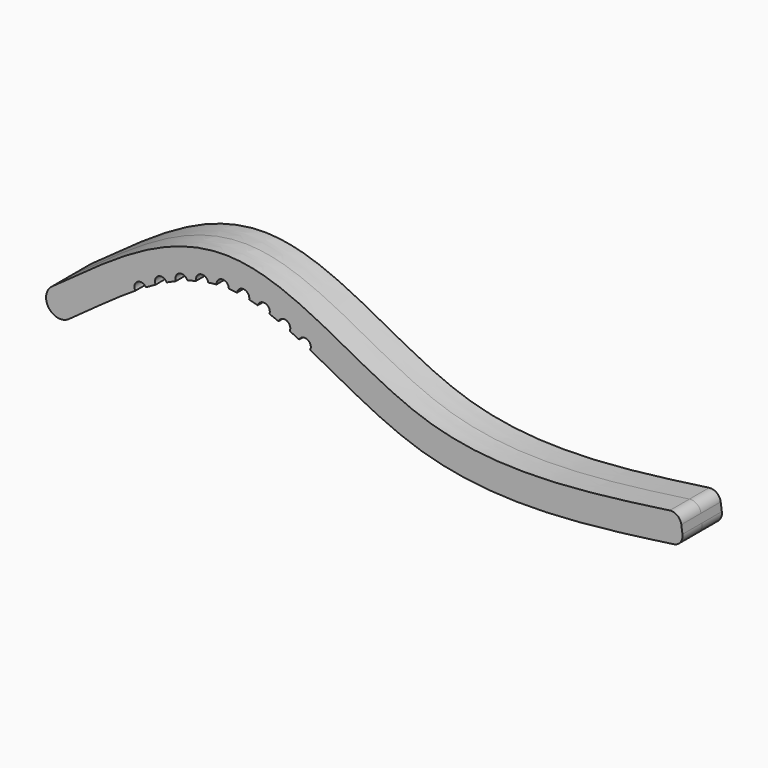
from build123d import *

# Parameters (mm, degrees)
F1_DEPTH = 6
F2_R     = 2.5
F3_R     = 1.5
F4_DEPTH = 12.0010001


# Not quite as in the source:
# - the dataset's text gives a spline's control points without its knots; the knots are read off the source's solid


with BuildPart() as f1:
    # F0 (on Front) → F1 (new body, symmetric)
    with BuildSketch(Plane.XZ):
        with BuildLine():
            ThreePointArc((-4.0449113911, 5.7130282546), (-4.8789698229, 0.8340584318), (0, 0))
            add(Edge.make_bspline(
                [(0, 0), (12.6866183221, 8.9823198273), (39.097046681, 31.0254585121), (84.6231120805, -9.3204370609), (127.451649596, -3.1579744512), (150, 0)],
                knots=[0, 0, 0, 0, 0.3024009423, 0.6287352131, 1, 1, 1, 1], degree=3))
            Line((150, 0), (149.0291016229, 6.9323413319))
            add(Edge.make_bspline(
                [(-4.0449113911, 5.7130282546), (-1.4893265055, 7.522421444), (2.4289578755, 10.3991251109), (7.8311540893, 14.2258677584), (11.985518828, 17.0073967049), (16.2624014486, 19.6143417246), (20.6904437749, 21.9553087459), (25.3048430013, 23.9276125636), (29.3354802395, 25.1619067391), (32.6783528938, 25.828942319), (35.2427144442, 26.1479585874), (37.419626365, 26.2456905562), (39.1857443489, 26.2125714545), (40.9384858731, 26.1049312213), (43.0954900321, 25.8409787708), (46.4720299209, 25.1788075072), (50.5545204313, 23.9683165065), (55.2777949463, 22.0808731164), (59.8806691618, 19.8983979978), (64.4079741748, 17.5399643684), (68.8916038218, 15.1143270568), (73.3515183232, 12.7253635973), (77.7977758185, 10.4736185968), (81.4936492304, 8.7918611912), (84.4432333572, 7.608120023), (86.2840306834, 6.9438576049), (87.7535671011, 6.4632867232), (89.2383433444, 6.0114309597), (91.1197744412, 5.5000916427), (93.4192059549, 4.9686735981), (96.5398637001, 4.3656966777), (100.5419436116, 3.8023805188), (105.4978361754, 3.4066907033), (110.5952082283, 3.2657358671), (117.5618909593, 3.3809979789), (126.5522503494, 4.0218977706), (137.6717582852, 5.3370647038), (145.2302773967, 6.4003028618), (149.0291016229, 6.9323413319)],
                knots=[0, 0, 0, 0, 0.0625, 0.09375, 0.125, 0.15625, 0.1875, 0.21875, 0.25, 0.265625, 0.28125, 0.296875, 0.3046875, 0.3125, 0.328125, 0.34375, 0.375, 0.40625, 0.4375, 0.46875, 0.5, 0.53125, 0.5625, 0.59375, 0.609375, 0.625, 0.6328125, 0.640625, 0.65625, 0.671875, 0.6875, 0.71875, 0.75, 0.78125, 0.8125, 0.875, 0.9375, 1, 1, 1, 1], degree=3))
        make_face()
    extrude(amount=F1_DEPTH, both=True)

    # F2
    f2_edges = [f1.edges().sort_by_distance(p)[0] for p in [
        (149.029102, 3, 6.932341),
        (150, 3, 0),
        (149.029102, -3, 6.932341),
        (150, -3, 0),
    ]]
    fillet(f2_edges, radius=F2_R)

    # F3 (on face) → F4 (cut, through all)
    with BuildSketch(Plane.XZ.offset(6)):
        with Locations((37.5310791936, 19.2248344713)):
            Circle(F3_R)
        with Locations((32.5310791936, 18.6530319414)):
            Circle(F3_R)
        with Locations((27.5310791936, 17.192316528)):
            Circle(F3_R)
        with Locations((22.5310791936, 14.983407983)):
            Circle(F3_R)
        with Locations((17.5310791936, 12.1773542976)):
            Circle(F3_R)
        with Locations((42.5310791936, 18.806197108)):
            Circle(F3_R)
        with Locations((47.5310791936, 17.51930095)):
            Circle(F3_R)
        with Locations((52.5310791936, 15.5840389676)):
            Circle(F3_R)
        with Locations((57.5310791936, 13.2102312001)):
            Circle(F3_R)
    extrude(amount=-F4_DEPTH, mode=Mode.SUBTRACT)


with BuildPart() as f5_1:
    # F5: copy of F1
    add(f1.part)


with BuildPart() as f6_1:
    # F6: copy of F1
    add(f1.part)


solid = Compound([f1.part, f6_1.part])
